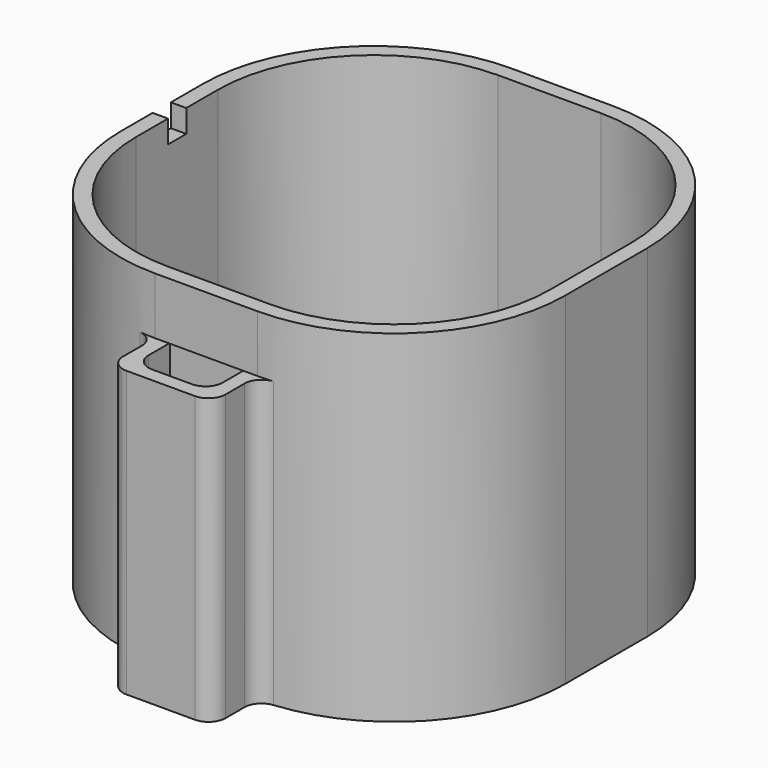
from build123d import *

# Parameters (mm, degrees)
F0_W      = 78
F0_H      = 78
F1_DEPTH  = 60
F2_R      = 30
F4_T      = -2.7
F3_W      = 18
F3_H      = 10
F5_DEPTH  = 25
F6_DEPTH  = 50
F7_T      = -2.5
F8_R      = 5.5856812821
F9_DEPTH  = 25
F10_R     = 3
F11_W     = 2.7
F11_H     = 4
F12_DEPTH = 4


# Not quite as in the source:
# - a shell that OpenCascade refuses in one call is made with other operations: the cavity is built on its own and cut out


with BuildPart() as f1:
    # F0 (on Top) → F1 (new body)
    with BuildSketch(Plane.XY):
        Rectangle(F0_W, F0_H)
    extrude(amount=F1_DEPTH)

    # F2
    f2_edges = [f1.edges().sort_by_distance(p)[0] for p in [
        (-39, -39, 30),
        (39, -39, 30),
        (39, 39, 30),
        (-39, 39, 30),
    ]]
    fillet(f2_edges, radius=F2_R)

    # F4
    f4_openings = [f1.faces().sort_by_distance(p)[0] for p in [
        (0, 0, 60),
    ]]
    offset(amount=F4_T, openings=f4_openings)

    # F3 (on Top) → F5 (cut)
    with BuildSketch(Plane.XY):
        with Locations((0, -44)):
            Rectangle(F3_W, F3_H)
    extrude(amount=-F5_DEPTH, mode=Mode.SUBTRACT)

    # F3 (on Top) → F6 (join)
    with BuildSketch(Plane.XY):
        with Locations((0, -44)):
            Rectangle(F3_W, F3_H)
    extrude(amount=F6_DEPTH)

    # F7: a shell. OpenCascade refuses it in one call, so the cavity is built on its own and cut out:
    # the body offset inwards by the wall thickness, plus a prism from it out through each open face.
    f7_core = offset(f1.part, amount=F7_T, kind=Kind.INTERSECTION, mode=Mode.PRIVATE)
    f7_exits = [f7_core.faces().sort_by_distance(p)[0] for p in [
        (0, -42.65, 47.5),
    ]]
    add(f7_core, mode=Mode.SUBTRACT)
    extrude(f7_exits, amount=-F7_T, mode=Mode.SUBTRACT)

    # F8 (on face) → F9 (cut)
    with BuildSketch(Plane.XZ.offset(39)):
        with Locations((0, 10.1356906816)):
            Circle(F8_R)
    extrude(amount=-F9_DEPTH, mode=Mode.SUBTRACT)

    # F10
    f10_edges = [f1.edges().sort_by_distance(p)[0] for p in [
        (-9, -49, 25),
        (9, -49, 25),
        (-6.5, -46.5, 26.25),
        (6.5, -46.5, 26.25),
        (-9, -39, 25),
        (-9, -39, 55),
        (9, -39, 25),
        (9, -39, 55),
    ]]
    fillet(f10_edges, radius=F10_R)

    # F11 (on face) → F12 (cut)
    with BuildSketch(Plane.XY.offset(60)):
        with Locations((-37.65, 0)):
            Rectangle(F11_W, F11_H)
    extrude(amount=-F12_DEPTH, mode=Mode.SUBTRACT)


solid = f1.part
